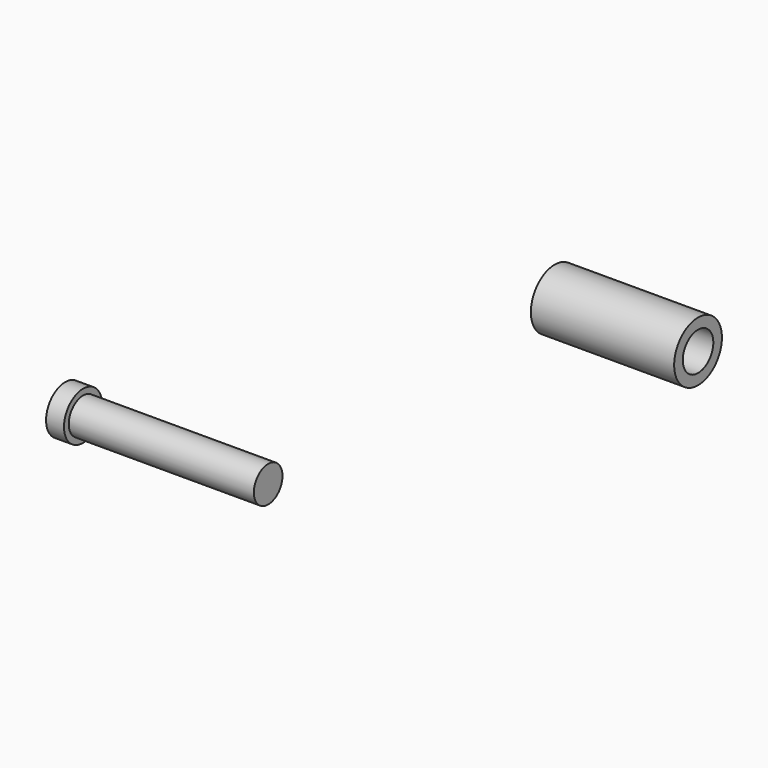
from build123d import *

# Parameters (mm, degrees)
F1_R     = 2.5
F1_R_2   = 1.6
F2_DEPTH = 12
F4_R     = 2.05
F4_R_2   = 1.6
F5_DEPTH = 1.5


with BuildPart() as f2:
    # F1 (on Right) → F2 (new body)
    with BuildSketch(Plane.YZ):
        with Locations((30, 0)):
            Circle(F1_R)
        with Locations((30, 0)):
            Circle(F1_R_2, mode=Mode.SUBTRACT)
    extrude(amount=F2_DEPTH)

    # F4 (on face) → F5 (cut)
    with BuildSketch(Plane(origin=(0, 0, 0), x_dir=(0, -1, 0), z_dir=(-1, 0, 0))):
        with Locations((-30, 0)):
            Circle(F4_R)
        with Locations((-30, 0)):
            Circle(F4_R_2, mode=Mode.SUBTRACT)
        with Locations((-30, 0)):
            Circle(F4_R_2)
    extrude(amount=-F5_DEPTH, mode=Mode.SUBTRACT)


with BuildPart() as f3:
    # F0 (on Front) → F3 (revolve)
    with BuildSketch(Plane.XZ):
        Polygon((0, -1.5), (0, 0), (-15.5, 0), (-15.5, 0.5), (-17, 0.5), (-17, -1.5), align=None)
    revolve(axis=Axis((-8.5, 0, -1.5), (1, 0, 0)))


solid = Compound([f2.part, f3.part])
